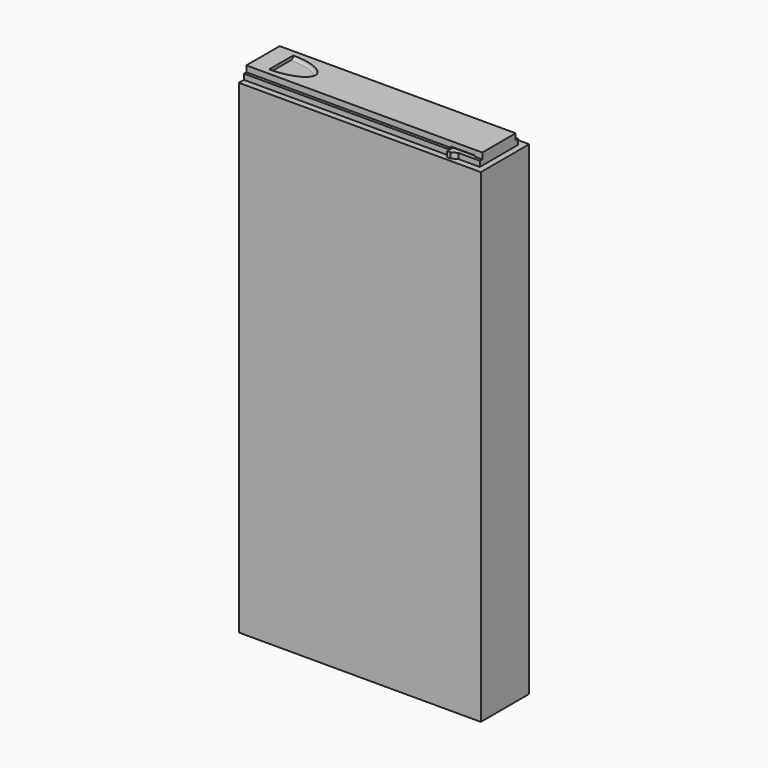
from build123d import *

# Parameters (mm, degrees)
F0_W      = 40
F0_H      = 10
F1_DEPTH  = 80
F3_START  = -2
F2_W      = 33
F2_H      = 8
F3_DEPTH  = 77
F5_START  = -2
F4_R      = 1.5
F5_DEPTH  = 28
F7_DEPTH  = 39
F9_START  = -1
F8_W      = 0.5
F8_H      = 1
F9_DEPTH  = 38
F11_DEPTH = 0.9
F12_W     = 39
F12_H     = 6.9
F13_DEPTH = 1
F14_W     = 3.9498324515
F14_H     = 0.2
F15_DEPTH = 1.2
F16_W     = 3.95
F16_H     = 0.2
F17_DEPTH = 1.2
F19_DEPTH = 0.5
F20_R     = 0.49999


# Not quite as in the source:
# - a fillet or chamfer is up to 0.001 mm smaller than in the source, because OpenCascade refuses the exact size


with BuildPart() as f1:
    # F0 (on Top) → F1 (new body)
    with BuildSketch(Plane.XY):
        Rectangle(F0_W, F0_H)
    extrude(amount=F1_DEPTH)

    # F2 (on face) → F3 (cut)
    with BuildSketch(Plane.XY.offset(80).offset(F3_START)):
        with Locations((2.5, 0)):
            Rectangle(F2_W, F2_H)
    extrude(amount=-F3_DEPTH, mode=Mode.SUBTRACT)

    # F4 (on face) → F5 (cut)
    with BuildSketch(Plane.XY.offset(80).offset(F5_START)):
        with Locations((-17, 0)):
            Circle(F4_R)
    extrude(amount=-F5_DEPTH, mode=Mode.SUBTRACT)

    # F6 (on face) → F7 (cut)
    with BuildSketch(Plane(origin=(-20, 0, 0), x_dir=(0, -1, 0), z_dir=(-1, 0, 0))):
        Polygon((3.5, 79), (3.5, 80), (-3.5, 80), (-3.5, 79), (-4, 79), (-4, 78), (4, 78), (4, 79), align=None)
    extrude(amount=-F7_DEPTH, mode=Mode.SUBTRACT)

    # F8 (on face) → F9 (cut)
    with BuildSketch(Plane(origin=(-20, 0, 0), x_dir=(0, -1, 0), z_dir=(-1, 0, 0)).offset(F9_START)):
        with Locations((4.25, 78.5)):
            Rectangle(F8_W, F8_H)
        with Locations((-4.25, 78.5)):
            Rectangle(F8_W, F8_H)
    extrude(amount=-F9_DEPTH, mode=Mode.SUBTRACT)


with BuildPart() as f11:
    # F10 (on face) → F11 (new body)
    with BuildSketch(Plane.XY.offset(80)):
        with BuildLine():
            Line((19, -3.95), (19, -3.5))
            Line((19, -3.5), (19, 3.5))
            Line((19, 3.5), (19, 3.95))
            Line((19, 3.95), (15.5, 3.95))
            Line((15.5, 3.95), (14.5909090909, 4.45))
            Line((14.5909090909, 4.45), (14, 4.45))
            Line((14, 4.45), (14, 3.95))
            Line((14, 3.95), (14, 3.5000000002))
            Line((14, 3.5000000002), (13.9999991525, 3.25))
            Line((13.9999991525, 3.25), (17.25, 3.25))
            ThreePointArc((17.25, 3.25), (17.75, 2.75), (17.25, 2.25))
            Line((17.25, 2.25), (13.8, 2.25))
            Line((13.8, 2.25), (13.8, 3.5))
            Line((13.8, 3.5), (13.8, 3.95))
            Line((13.8, 3.95), (-20, 3.95))
            Line((-20, 3.95), (-20, -3.95))
            Line((-20, -3.95), (13.8, -3.95))
            Line((13.8, -3.95), (13.8, -3.5))
            Line((13.8, -3.5), (13.8, -2.25))
            Line((13.8, -2.25), (17.2498324515, -2.25))
            ThreePointArc((17.2498324515, -2.25), (17.7498324515, -2.75), (17.2498324515, -3.25))
            Line((17.2498324515, -3.25), (13.9998308422, -3.25))
            Line((13.9998308422, -3.25), (14, -3.5))
            Line((14, -3.5), (14, -3.95))
            Line((14, -3.95), (14, -4.4487268106))
            Line((14, -4.4487268106), (14.5903386392, -4.4505964817))
            Line((14.5903386392, -4.4505964817), (15.5, -3.95))
            Line((15.5, -3.95), (19, -3.95))
        make_face()
    extrude(amount=F11_DEPTH)

    # F12 (on face) → F13 (join)
    with BuildSketch(Plane.XY.offset(80.9)):
        with Locations((-0.5, 0)):
            Rectangle(F12_W, F12_H)
    extrude(amount=F13_DEPTH)

    # F14 (on face) → F15 (cut)
    with BuildSketch(Plane.XZ.offset(3.45)):
        with Locations((15.7749162257, 81)):
            Rectangle(F14_W, F14_H)
    extrude(amount=-F15_DEPTH, mode=Mode.SUBTRACT)

    # F16 (on face) → F17 (cut)
    with BuildSketch(Plane(origin=(0, 3.45, 0), x_dir=(-1, 0, 0), z_dir=(0, 1, 0))):
        with Locations((-15.775, 81)):
            Rectangle(F16_W, F16_H)
    extrude(amount=-F17_DEPTH, mode=Mode.SUBTRACT)

    # F18 (on face) → F19 (cut)
    with BuildSketch(Plane.XY.offset(81.9)):
        with BuildLine():
            Line((-17, 2.5), (-17, 0))
            Line((-17, 0), (-17, -2.5))
            add(Edge.make_bspline(
                [(-17, -2.5), (-11.3068194012, -2.5), (-11.3068194012, 0), (-11.3068194012, 2.5), (-17, 2.5)],
                knots=[1.5707963268, 1.5707963268, 1.5707963268, 3.1415926536, 3.1415926536, 4.7123889804, 4.7123889804, 4.7123889804], degree=2, weights=[1, 0.7071067812, 1, 0.7071067812, 1]))
        make_face()
    extrude(amount=-F19_DEPTH, mode=Mode.SUBTRACT)

    # F20 (radius 0.5 in the source; OpenCascade refuses exactly that, so slightly less here)
    f20_edges = [f11.edges().sort_by_distance(p)[0] for p in [
        (-11.306819, 0, 81.4),
    ]]
    fillet(f20_edges, radius=F20_R)


solid = Compound([f1.part, f11.part])
